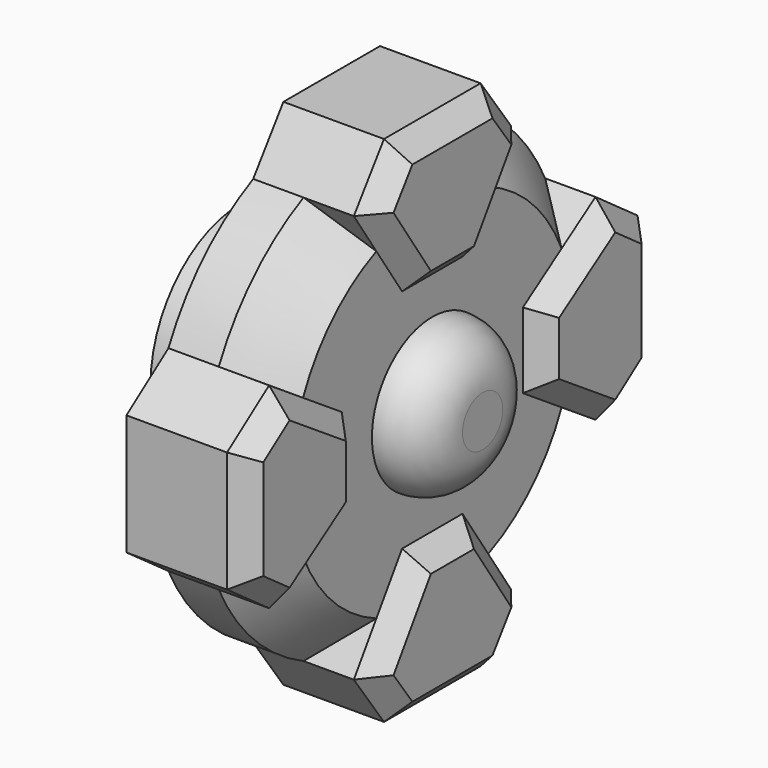
from build123d import *

# Parameters (mm, degrees)
F1_DEPTH = 10
F2_DEPTH = 12
F3_SIZE  = 5
F4_SIZE  = 1.99999
F5_R     = 7.5
F6_DEPTH = 5
F7_R     = 4.99999
F9_DEPTH = 9


# Not quite as in the source:
# - a fillet or chamfer is up to 0.001 mm smaller than in the source, because OpenCascade refuses the exact size
# - a feature names something its author has since deleted; it is built from what else it names


with BuildPart() as f1:
    # F0 (on Right) → F1 (new body)
    with BuildSketch(Plane.YZ):
        with BuildLine():
            Line((11.25, 3.75), (20.2777587519, 9.75))
            ThreePointArc((20.2777587519, 9.75), (15.9099025767, 15.9099025767), (9.75, 20.2777587519))
            Line((9.75, 20.2777587519), (3.75, 11.25))
            Line((3.75, 11.25), (0, 11.25))
            Line((0, 11.25), (-3.75, 11.25))
            Line((-3.75, 11.25), (-9.75, 20.2777587519))
            ThreePointArc((-9.75, 20.2777587519), (-15.9099025767, 15.9099025767), (-20.2777587519, 9.75))
            Line((-20.2777587519, 9.75), (-11.25, 3.75))
            Line((-11.25, 3.75), (-11.25, 0))
            Line((-11.25, 0), (-11.25, -3.75))
            Line((-11.25, -3.75), (-20.2777587519, -9.75))
            ThreePointArc((-20.2777587519, -9.75), (-15.9099025767, -15.9099025767), (-9.75, -20.2777587519))
            Line((-9.75, -20.2777587519), (-3.75, -11.25))
            Line((-3.75, -11.25), (0, -11.25))
            Line((0, -11.25), (3.75, -11.25))
            Line((3.75, -11.25), (9.75, -20.2777587519))
            ThreePointArc((9.75, -20.2777587519), (15.9099025767, -15.9099025767), (20.2777587519, -9.75))
            Line((20.2777587519, -9.75), (11.25, -3.75))
            Line((11.25, -3.75), (11.25, 0))
            Line((11.25, 0), (11.25, 3.75))
        make_face()
    extrude(amount=F1_DEPTH)

    # F0 (on Right) → F2 (join)
    with BuildSketch(Plane.YZ):
        with BuildLine():
            Line((3.75, 11.25), (9.75, 20.2777587519))
            ThreePointArc((9.75, 20.2777587519), (0, 22.5), (-9.75, 20.2777587519))
            Line((-9.75, 20.2777587519), (-3.75, 11.25))
            Line((-3.75, 11.25), (0, 11.25))
            Line((0, 11.25), (3.75, 11.25))
        make_face()
        with BuildLine():
            ThreePointArc((-9.75, 20.2777587519), (0, 22.5), (9.75, 20.2777587519))
            Line((9.75, 20.2777587519), (6, 25.5))
            Line((6, 25.5), (0, 25.5))
            Line((0, 25.5), (-6, 25.5))
            Line((-6, 25.5), (-9.75, 20.2777587519))
        make_face()
        with BuildLine():
            Line((-11.25, 3.75), (-20.2777587519, 9.75))
            ThreePointArc((-20.2777587519, 9.75), (-22.5, 0), (-20.2777587519, -9.75))
            Line((-20.2777587519, -9.75), (-11.25, -3.75))
            Line((-11.25, -3.75), (-11.25, 0))
            Line((-11.25, 0), (-11.25, 3.75))
        make_face()
        with BuildLine():
            ThreePointArc((-20.2777587519, -9.75), (-22.5, 0), (-20.2777587519, 9.75))
            Line((-20.2777587519, 9.75), (-25.5, 6))
            Line((-25.5, 6), (-25.5, 0))
            Line((-25.5, 0), (-25.5, -6))
            Line((-25.5, -6), (-20.2777587519, -9.75))
        make_face()
        with BuildLine():
            ThreePointArc((-9.75, -20.2777587519), (0, -22.5), (9.75, -20.2777587519))
            Line((9.75, -20.2777587519), (3.75, -11.25))
            Line((3.75, -11.25), (0, -11.25))
            Line((0, -11.25), (-3.75, -11.25))
            Line((-3.75, -11.25), (-9.75, -20.2777587519))
        make_face()
        with BuildLine():
            Line((6, -25.5), (9.75, -20.2777587519))
            ThreePointArc((9.75, -20.2777587519), (0, -22.5), (-9.75, -20.2777587519))
            Line((-9.75, -20.2777587519), (-6, -25.5))
            Line((-6, -25.5), (0, -25.5))
            Line((0, -25.5), (6, -25.5))
        make_face()
        with BuildLine():
            ThreePointArc((20.2777587519, -9.75), (21.93740609, -5.0000214041), (22.5, 0))
            ThreePointArc((22.5, 0), (21.93740609, 5.0000214041), (20.2777587519, 9.75))
            Line((20.2777587519, 9.75), (11.25, 3.75))
            Line((11.25, 3.75), (11.25, 0))
            Line((11.25, 0), (11.25, -3.75))
            Line((11.25, -3.75), (20.2777587519, -9.75))
        make_face()
        with BuildLine():
            ThreePointArc((20.2777587519, 9.75), (21.93740609, 5.0000214041), (22.5, 0))
            ThreePointArc((22.5, 0), (21.93740609, -5.0000214041), (20.2777587519, -9.75))
            Line((20.2777587519, -9.75), (25.5, -6))
            Line((25.5, -6), (25.5, 0))
            Line((25.5, 0), (25.5, 6))
            Line((25.5, 6), (20.2777587519, 9.75))
        make_face()
    extrude(amount=F2_DEPTH)

    # F3
    f3_edges = [f1.edges().sort_by_distance(p)[0] for p in [
        (10, 15.909903, 15.909903),
        (10, -15.909903, 15.909903),
        (10, -15.909903, -15.909903),
        (10, 15.909903, -15.909903),
    ]]
    chamfer(f3_edges, length=F3_SIZE)

    # F4 (size 2 in the source; OpenCascade refuses exactly that, so slightly less here)
    f4_edges = [f1.edges().sort_by_distance(p)[0] for p in [
        (12, 0, 25.5),
        (12, -7.875, 22.888879),
        (12, 7.875, 22.888879),
        (12, -6.75, 15.763879),
        (12, 6.75, 15.763879),
        (12, 0, 11.25),
        (12, -15.763879, 6.75),
        (12, -22.888879, 7.875),
        (12, -25.5, 0),
        (12, -22.888879, -7.875),
        (12, -15.763879, -6.75),
        (12, -11.25, 0),
        (12, 0, -11.25),
        (12, -6.75, -15.763879),
        (12, -7.875, -22.888879),
        (12, 6.75, -15.763879),
        (12, 0, -25.5),
        (12, 7.875, -22.888879),
        (12, 15.763879, -6.75),
        (12, 11.25, 0),
        (12, 15.763879, 6.75),
        (12, 22.888879, 7.875),
        (12, 25.5, 0),
        (12, 22.888879, -7.875),
    ]]
    chamfer(f4_edges, length=F4_SIZE)

    # F5 (on face) → F6 (join)
    with BuildSketch(Plane.YZ.offset(10)):
        Circle(F5_R)
    extrude(amount=F6_DEPTH)

    # F7 (radius 5 in the source; OpenCascade refuses exactly that, so slightly less here)
    f7_edges = [f1.edges().sort_by_distance(p)[0] for p in [
        (15, -7.5, 0),
    ]]
    fillet(f7_edges, radius=F7_R)

    # F8 (on face) → F9 (join)
    with BuildSketch(Plane.YZ):
        with BuildLine():
            ThreePointArc((0, -11.25), (7.9549512883, -7.9549512883), (11.25, 0))
            ThreePointArc((11.25, 0), (7.9549512883, 7.9549512883), (0, 11.25))
            ThreePointArc((0, 11.25), (-7.9549512883, 7.9549512883), (-11.25, 0))
            ThreePointArc((-11.25, 0), (-7.9549512883, -7.9549512883), (0, -11.25))
        make_face()
    extrude(amount=-F9_DEPTH)


solid = f1.part
